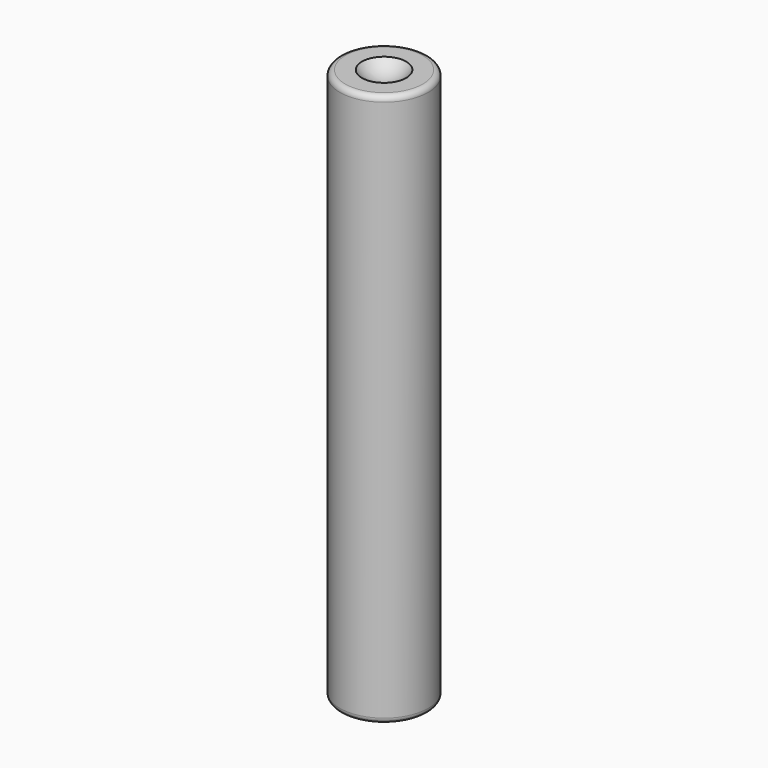
from build123d import *

# Parameters (mm, degrees)
F0_R          = 8
F1_DEPTH      = 50
F1_DEPTH_BACK = 50
F4_R          = 1


# Not quite as in the source:
# - a pattern or mirror of a feature is missing from the dataset's text; its kind, count and spacing are read off the source's solid


with BuildPart() as f1:
    # F0 (on Top) → F1 (new body, two sides)
    with BuildSketch(Plane.XY) as f1_sk:
        Circle(F0_R)
    extrude(amount=F1_DEPTH)
    extrude(f1_sk.sketch, amount=-F1_DEPTH_BACK)

    # F2 (on Front) → F3 (revolve, cut)
    with BuildSketch(Plane.XZ):
        with BuildLine():
            ThreePointArc((0, 58), (-5, 53), (0, 48))
            Line((0, 48), (0, 53))
            Line((0, 53), (0, 58))
        make_face()
    f3 = revolve(axis=Axis((0, 0, 53), (0, 0, -1)), mode=Mode.SUBTRACT)

    # F3_copies: F3 across plane
    add(f3.mirror(Plane(origin=(0, 0, 0), x_dir=(-1, 0, 0), z_dir=(0, 0, -1))), mode=Mode.SUBTRACT)

    # F4
    f4_edges = [f1.edges().sort_by_distance(p)[0] for p in [
        (-8, 0, 50),
        (-8, 0, -50),
    ]]
    fillet(f4_edges, radius=F4_R)


solid = f1.part
